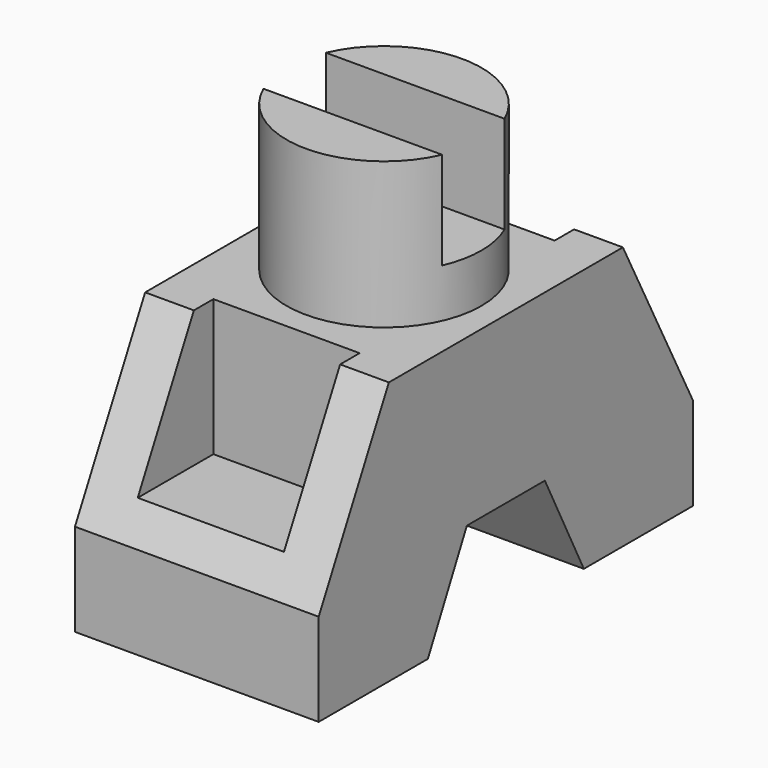
from build123d import *

# Parameters (mm, degrees)
F0_W      = 96
F0_H      = 54
F1_DEPTH  = 25
F2_SIZE2  = 35
F2_SIZE   = 18
F4_DEPTH  = 50.001
F5_R      = 20
F6_DEPTH  = 30
F7_W      = 40
F7_H      = 16
F8_DEPTH  = 20
F9_W      = 30
F9_H      = 28
F10_DEPTH = 23


# Not quite as in the source:
# - a pattern or mirror of a feature is missing from the dataset's text; its kind, count and spacing are read off the source's solid


with BuildPart() as f1:
    # F0 (on Right) → F1 (new body, symmetric)
    with BuildSketch(Plane.YZ):
        Rectangle(F0_W, F0_H)
    extrude(amount=F1_DEPTH, both=True)

    # F2
    f2_edges = [f1.edges().sort_by_distance(p)[0] for p in [
        (0, -48, 27),
        (0, 48, 27),
    ]]
    f2_side = f1.faces().sort_by_distance((0, 0, 27))[0]
    chamfer(f2_edges, length=F2_SIZE, length2=F2_SIZE2, reference=f2_side)

    # F3 (on face) → F4 (cut, through all)
    with BuildSketch(Plane.YZ.offset(25)):
        Polygon((-10, -7), (-20, -27), (20, -27), (10, -7), align=None)
    extrude(amount=-F4_DEPTH, mode=Mode.SUBTRACT)

    # F5 (on face) → F6 (join)
    with BuildSketch(Plane.XY.offset(27)):
        Circle(F5_R)
    extrude(amount=F6_DEPTH)

    # F7 (on face) → F8 (cut)
    with BuildSketch(Plane.XY.offset(57)):
        Rectangle(F7_W, F7_H)
    extrude(amount=-F8_DEPTH, mode=Mode.SUBTRACT)

    # F9 (on face) → F10 (cut)
    with BuildSketch(Plane.XZ.offset(48)):
        with Locations((0, 13)):
            Rectangle(F9_W, F9_H)
    f10 = extrude(amount=-F10_DEPTH, mode=Mode.SUBTRACT)

    # F10_copies: F10 across plane
    add(f10.mirror(Plane.ZX), mode=Mode.SUBTRACT)


solid = f1.part
